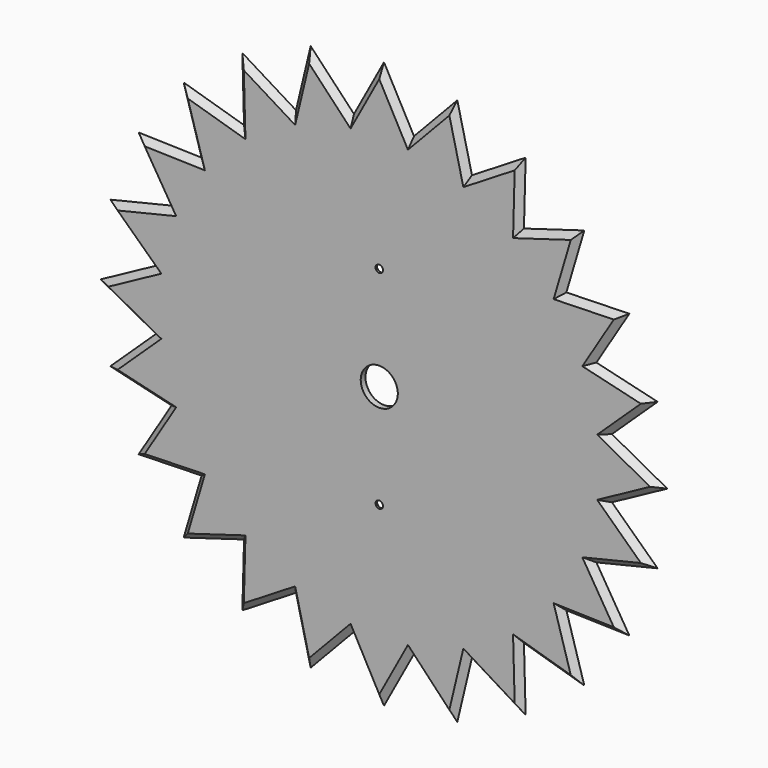
from build123d import *

# Parameters (mm, degrees)
F1_DEPTH       = 5.08
F2_SIZE        = 5.07999
F4_D           = 6.35
F4_CSINK_D     = 13.208
F4_CSINK_ANGLE = 90
F5_R           = 15.875
F6_DEPTH       = 25.4


# Not quite as in the source:
# - a fillet or chamfer is up to 0.001 mm smaller than in the source, because OpenCascade refuses the exact size


with BuildPart() as f1:
    # F0 (on Front) → F1 (new body)
    with BuildSketch(Plane.XZ):
        with BuildLine():
            ThreePointArc((181.8656859748, 75.3312336611), (190.142498905, 50.9485290284), (195.1659209614, 25.6940809385))
            Line((195.1659209614, 25.6940809385), (234.3046276829, 62.7817357705))
            Line((234.3046276829, 62.7817357705), (181.8656859748, 75.3312336611))
        make_face()
        with BuildLine():
            ThreePointArc((156.1716050363, 119.8346873004), (170.477100735, 98.425), (181.8656859748, 75.3312336611))
            Line((181.8656859748, 75.3312336611), (210.071782196, 121.285))
            Line((210.071782196, 121.285), (156.1716050363, 119.8346873004))
        make_face()
        with BuildLine():
            ThreePointArc((119.8346873004, 156.1716050363), (139.1939698766, 139.1939698766), (156.1716050363, 119.8346873004))
            Line((156.1716050363, 119.8346873004), (171.5228919124, 171.5228919124))
            Line((171.5228919124, 171.5228919124), (119.8346873004, 156.1716050363))
        make_face()
        with BuildLine():
            ThreePointArc((75.3312336611, 181.8656859748), (98.425, 170.477100735), (119.8346873004, 156.1716050363))
            Line((119.8346873004, 156.1716050363), (121.285, 210.071782196))
            Line((121.285, 210.071782196), (75.3312336611, 181.8656859748))
        make_face()
        with BuildLine():
            ThreePointArc((25.6940809385, 195.1659209614), (50.9485290284, 190.142498905), (75.3312336611, 181.8656859748))
            Line((75.3312336611, 181.8656859748), (62.7817357705, 234.3046276829))
            Line((62.7817357705, 234.3046276829), (25.6940809385, 195.1659209614))
        make_face()
        with BuildLine():
            ThreePointArc((-25.6940809385, 195.1659209614), (0, 196.85), (25.6940809385, 195.1659209614))
            Line((25.6940809385, 195.1659209614), (0, 242.57))
            Line((0, 242.57), (-25.6940809385, 195.1659209614))
        make_face()
        with BuildLine():
            ThreePointArc((-75.3312336611, 181.8656859748), (-50.9485290284, 190.142498905), (-25.6940809385, 195.1659209614))
            Line((-25.6940809385, 195.1659209614), (-62.7817357705, 234.3046276829))
            Line((-62.7817357705, 234.3046276829), (-75.3312336611, 181.8656859748))
        make_face()
        with BuildLine():
            ThreePointArc((-119.8346873004, 156.1716050363), (-98.425, 170.477100735), (-75.3312336611, 181.8656859748))
            Line((-75.3312336611, 181.8656859748), (-121.285, 210.071782196))
            Line((-121.285, 210.071782196), (-119.8346873004, 156.1716050363))
        make_face()
        with BuildLine():
            ThreePointArc((-156.1716050363, 119.8346873004), (-139.1939698766, 139.1939698766), (-119.8346873004, 156.1716050363))
            Line((-119.8346873004, 156.1716050363), (-171.5228919124, 171.5228919124))
            Line((-171.5228919124, 171.5228919124), (-156.1716050363, 119.8346873004))
        make_face()
        with BuildLine():
            ThreePointArc((-181.8656859748, 75.3312336611), (-170.477100735, 98.425), (-156.1716050363, 119.8346873004))
            Line((-156.1716050363, 119.8346873004), (-210.071782196, 121.285))
            Line((-210.071782196, 121.285), (-181.8656859748, 75.3312336611))
        make_face()
        with BuildLine():
            ThreePointArc((-195.1659209614, 25.6940809385), (-190.142498905, 50.9485290284), (-181.8656859748, 75.3312336611))
            Line((-181.8656859748, 75.3312336611), (-234.3046276829, 62.7817357705))
            Line((-234.3046276829, 62.7817357705), (-195.1659209614, 25.6940809385))
        make_face()
        with BuildLine():
            ThreePointArc((-195.1659209614, -25.6940809385), (-196.85, 0), (-195.1659209614, 25.6940809385))
            Line((-195.1659209614, 25.6940809385), (-242.57, 0))
            Line((-242.57, 0), (-195.1659209614, -25.6940809385))
        make_face()
        with BuildLine():
            Line((-234.3046276829, -62.7817357705), (-181.8656859748, -75.3312336611))
            ThreePointArc((-181.8656859748, -75.3312336611), (-190.142498905, -50.9485290284), (-195.1659209614, -25.6940809385))
            Line((-195.1659209614, -25.6940809385), (-234.3046276829, -62.7817357705))
        make_face()
        with BuildLine():
            Line((-210.071782196, -121.285), (-156.1716050363, -119.8346873004))
            ThreePointArc((-156.1716050363, -119.8346873004), (-170.477100735, -98.425), (-181.8656859748, -75.3312336611))
            Line((-181.8656859748, -75.3312336611), (-210.071782196, -121.285))
        make_face()
        with BuildLine():
            Line((-171.5228919124, -171.5228919124), (-119.8346873004, -156.1716050363))
            ThreePointArc((-119.8346873004, -156.1716050363), (-139.1939698766, -139.1939698766), (-156.1716050363, -119.8346873004))
            Line((-156.1716050363, -119.8346873004), (-171.5228919124, -171.5228919124))
        make_face()
        with BuildLine():
            Line((-121.285, -210.071782196), (-75.3312336611, -181.8656859748))
            ThreePointArc((-75.3312336611, -181.8656859748), (-98.425, -170.477100735), (-119.8346873004, -156.1716050363))
            Line((-119.8346873004, -156.1716050363), (-121.285, -210.071782196))
        make_face()
        with BuildLine():
            Line((-62.7817357705, -234.3046276829), (-25.6940809385, -195.1659209614))
            ThreePointArc((-25.6940809385, -195.1659209614), (-50.9485290284, -190.142498905), (-75.3312336611, -181.8656859748))
            Line((-75.3312336611, -181.8656859748), (-62.7817357705, -234.3046276829))
        make_face()
        with BuildLine():
            Line((0, -242.57), (25.6940809385, -195.1659209614))
            ThreePointArc((25.6940809385, -195.1659209614), (0, -196.85), (-25.6940809385, -195.1659209614))
            Line((-25.6940809385, -195.1659209614), (0, -242.57))
        make_face()
        with BuildLine():
            Line((62.7817357705, -234.3046276829), (75.3312336611, -181.8656859748))
            ThreePointArc((75.3312336611, -181.8656859748), (50.9485290284, -190.142498905), (25.6940809385, -195.1659209614))
            Line((25.6940809385, -195.1659209614), (62.7817357705, -234.3046276829))
        make_face()
        with BuildLine():
            Line((121.285, -210.071782196), (119.8346873004, -156.1716050363))
            ThreePointArc((119.8346873004, -156.1716050363), (98.425, -170.477100735), (75.3312336611, -181.8656859748))
            Line((75.3312336611, -181.8656859748), (121.285, -210.071782196))
        make_face()
        with BuildLine():
            Line((171.5228919124, -171.5228919124), (156.1716050363, -119.8346873004))
            ThreePointArc((156.1716050363, -119.8346873004), (139.1939698766, -139.1939698766), (119.8346873004, -156.1716050363))
            Line((119.8346873004, -156.1716050363), (171.5228919124, -171.5228919124))
        make_face()
        with BuildLine():
            Line((210.071782196, -121.285), (181.8656859748, -75.3312336611))
            ThreePointArc((181.8656859748, -75.3312336611), (170.477100735, -98.425), (156.1716050363, -119.8346873004))
            Line((156.1716050363, -119.8346873004), (210.071782196, -121.285))
        make_face()
        with BuildLine():
            Line((234.3046276829, -62.7817357705), (195.1659209614, -25.6940809385))
            ThreePointArc((195.1659209614, -25.6940809385), (190.142498905, -50.9485290284), (181.8656859748, -75.3312336611))
            Line((181.8656859748, -75.3312336611), (234.3046276829, -62.7817357705))
        make_face()
        with BuildLine():
            ThreePointArc((195.1659209614, 25.6940809385), (196.4285290395, 12.874605989), (196.85, 0))
            ThreePointArc((196.85, 0), (196.4285290395, -12.874605989), (195.1659209614, -25.6940809385))
            Line((195.1659209614, -25.6940809385), (242.57, 0))
            Line((242.57, 0), (195.1659209614, 25.6940809385))
        make_face()
        with BuildLine():
            ThreePointArc((195.1659209614, -25.6940809385), (196.4285290395, -12.874605989), (196.85, 0))
            ThreePointArc((196.85, 0), (196.4285290395, 12.874605989), (195.1659209614, 25.6940809385))
            ThreePointArc((195.1659209614, 25.6940809385), (190.142498905, 50.9485290284), (181.8656859748, 75.3312336611))
            ThreePointArc((181.8656859748, 75.3312336611), (170.477100735, 98.425), (156.1716050363, 119.8346873004))
            ThreePointArc((156.1716050363, 119.8346873004), (139.1939698766, 139.1939698766), (119.8346873004, 156.1716050363))
            ThreePointArc((119.8346873004, 156.1716050363), (98.425, 170.477100735), (75.3312336611, 181.8656859748))
            ThreePointArc((75.3312336611, 181.8656859748), (50.9485290284, 190.142498905), (25.6940809385, 195.1659209614))
            ThreePointArc((25.6940809385, 195.1659209614), (0, 196.85), (-25.6940809385, 195.1659209614))
            ThreePointArc((-25.6940809385, 195.1659209614), (-50.9485290284, 190.142498905), (-75.3312336611, 181.8656859748))
            ThreePointArc((-75.3312336611, 181.8656859748), (-98.425, 170.477100735), (-119.8346873004, 156.1716050363))
            ThreePointArc((-119.8346873004, 156.1716050363), (-139.1939698766, 139.1939698766), (-156.1716050363, 119.8346873004))
            ThreePointArc((-156.1716050363, 119.8346873004), (-170.477100735, 98.425), (-181.8656859748, 75.3312336611))
            ThreePointArc((-181.8656859748, 75.3312336611), (-190.142498905, 50.9485290284), (-195.1659209614, 25.6940809385))
            ThreePointArc((-195.1659209614, 25.6940809385), (-196.85, 0), (-195.1659209614, -25.6940809385))
            ThreePointArc((-195.1659209614, -25.6940809385), (-190.142498905, -50.9485290284), (-181.8656859748, -75.3312336611))
            ThreePointArc((-181.8656859748, -75.3312336611), (-170.477100735, -98.425), (-156.1716050363, -119.8346873004))
            ThreePointArc((-156.1716050363, -119.8346873004), (-139.1939698766, -139.1939698766), (-119.8346873004, -156.1716050363))
            ThreePointArc((-119.8346873004, -156.1716050363), (-98.425, -170.477100735), (-75.3312336611, -181.8656859748))
            ThreePointArc((-75.3312336611, -181.8656859748), (-50.9485290284, -190.142498905), (-25.6940809385, -195.1659209614))
            ThreePointArc((-25.6940809385, -195.1659209614), (0, -196.85), (25.6940809385, -195.1659209614))
            ThreePointArc((25.6940809385, -195.1659209614), (50.9485290284, -190.142498905), (75.3312336611, -181.8656859748))
            ThreePointArc((75.3312336611, -181.8656859748), (98.425, -170.477100735), (119.8346873004, -156.1716050363))
            ThreePointArc((119.8346873004, -156.1716050363), (139.1939698766, -139.1939698766), (156.1716050363, -119.8346873004))
            ThreePointArc((156.1716050363, -119.8346873004), (170.477100735, -98.425), (181.8656859748, -75.3312336611))
            ThreePointArc((181.8656859748, -75.3312336611), (190.142498905, -50.9485290284), (195.1659209614, -25.6940809385))
        make_face()
    extrude(amount=F1_DEPTH)

    # F2 (size 5.08 in the source; OpenCascade refuses exactly that, so slightly less here)
    f2_edges = [f1.edges().sort_by_distance(p)[0] for p in [
        (208.085157, -5.08, 69.056485),
        (195.968734, -5.08, 98.308117),
        (183.121694, -5.08, 120.559844),
        (163.847248, -5.08, 145.67879),
        (145.67879, -5.08, 163.847248),
        (120.559844, -5.08, 183.121694),
        (98.308117, -5.08, 195.968734),
        (69.056485, -5.08, 208.085157),
        (44.237908, -5.08, 214.735274),
        (12.84704, -5.08, 218.86796),
        (-12.84704, -5.08, 218.86796),
        (-44.237908, -5.08, 214.735274),
        (-69.056485, -5.08, 208.085157),
        (-98.308117, -5.08, 195.968734),
        (-120.559844, -5.08, 183.121694),
        (-145.67879, -5.08, 163.847248),
        (-163.847248, -5.08, 145.67879),
        (-183.121694, -5.08, 120.559844),
        (-195.968734, -5.08, 98.308117),
        (-208.085157, -5.08, 69.056485),
        (-214.735274, -5.08, 44.237908),
        (-218.86796, -5.08, 12.84704),
        (-218.86796, -5.08, -12.84704),
        (-214.735274, -5.08, -44.237908),
        (-208.085157, -5.08, -69.056485),
        (-195.968734, -5.08, -98.308117),
        (-183.121694, -5.08, -120.559844),
        (-163.847248, -5.08, -145.67879),
        (-145.67879, -5.08, -163.847248),
        (-120.559844, -5.08, -183.121694),
        (-98.308117, -5.08, -195.968734),
        (-69.056485, -5.08, -208.085157),
        (-44.237908, -5.08, -214.735274),
        (-12.84704, -5.08, -218.86796),
        (12.84704, -5.08, -218.86796),
        (44.237908, -5.08, -214.735274),
        (69.056485, -5.08, -208.085157),
        (98.308117, -5.08, -195.968734),
        (120.559844, -5.08, -183.121694),
        (145.67879, -5.08, -163.847248),
        (163.847248, -5.08, -145.67879),
        (183.121694, -5.08, -120.559844),
        (195.968734, -5.08, -98.308117),
        (208.085157, -5.08, -69.056485),
        (214.735274, -5.08, -44.237908),
        (218.86796, -5.08, -12.84704),
        (218.86796, -5.08, 12.84704),
        (214.735274, -5.08, 44.237908),
    ]]
    chamfer(f2_edges, length=F2_SIZE)

    # F4 (through all)
    with Locations(Plane(origin=(0, 0, 0), x_dir=(-1, 0, 0), z_dir=(0, 1, 0))):
        with Locations((0, 88.9), (0, -88.9)):
            CounterSinkHole(F4_D / 2, F4_CSINK_D / 2, counter_sink_angle=F4_CSINK_ANGLE)

    # F5 (on face) → F6 (cut)
    with BuildSketch(Plane(origin=(0, 0, 0), x_dir=(-1, 0, 0), z_dir=(0, 1, 0))):
        Circle(F5_R)
    extrude(amount=-F6_DEPTH, mode=Mode.SUBTRACT)


solid = f1.part
